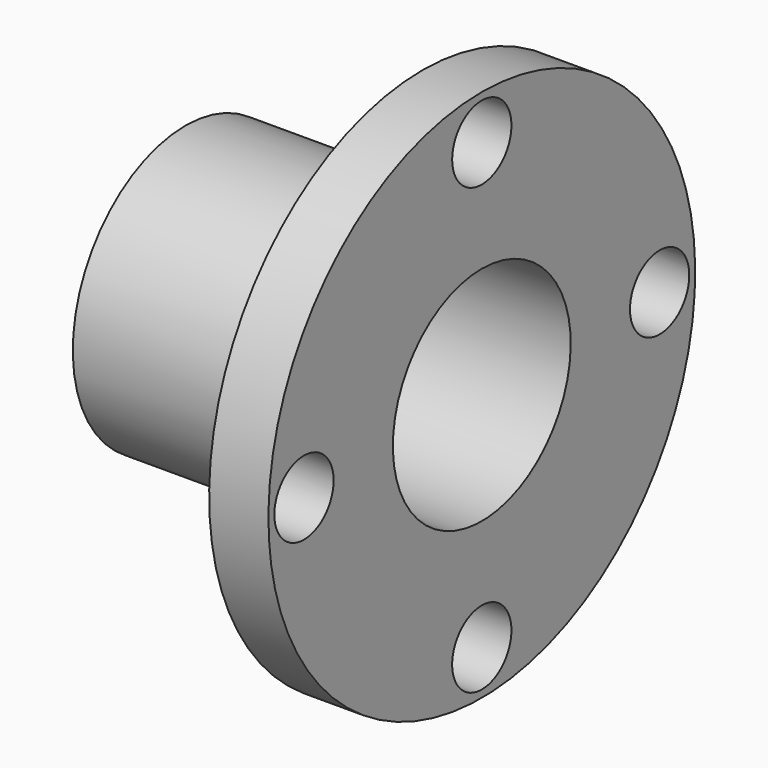
from build123d import *

# Parameters (mm, degrees)
F2_R            = 12.5
F3_DEPTH        = 281
F3_COPIES_COUNT = 4


# Not quite as in the source:
# - a pattern or mirror of a feature is missing from the dataset's text; its kind, count and spacing are read off the source's solid


with BuildPart() as f1:
    # F0 (on Front) → F1 (revolve)
    with BuildSketch(Plane.XZ):
        Polygon((-100, 37.5), (0, 37.5), (0, 90), (-20, 90), (-20, 47.5), (-100, 47.5), align=None)
    revolve(axis=Axis((-60.572553426, 0, 0), (1, 0, 0)))

    # F2 (on face) → F3 (cut)
    with BuildSketch(Plane(origin=(-20, 0, 0), x_dir=(0, -1, 0), z_dir=(-1, 0, 0))):
        with Locations((0, 75)):
            Circle(F2_R)
    f3 = extrude(amount=-F3_DEPTH, mode=Mode.SUBTRACT)

    # F3_copies: F3 ×4 about axis
    f3_copies_axis = Axis((0, 0, 0), (1, 0, 0))
    for i in range(1, F3_COPIES_COUNT):
        add(f3.rotate(f3_copies_axis, i * 360 / F3_COPIES_COUNT), mode=Mode.SUBTRACT)


solid = f1.part
